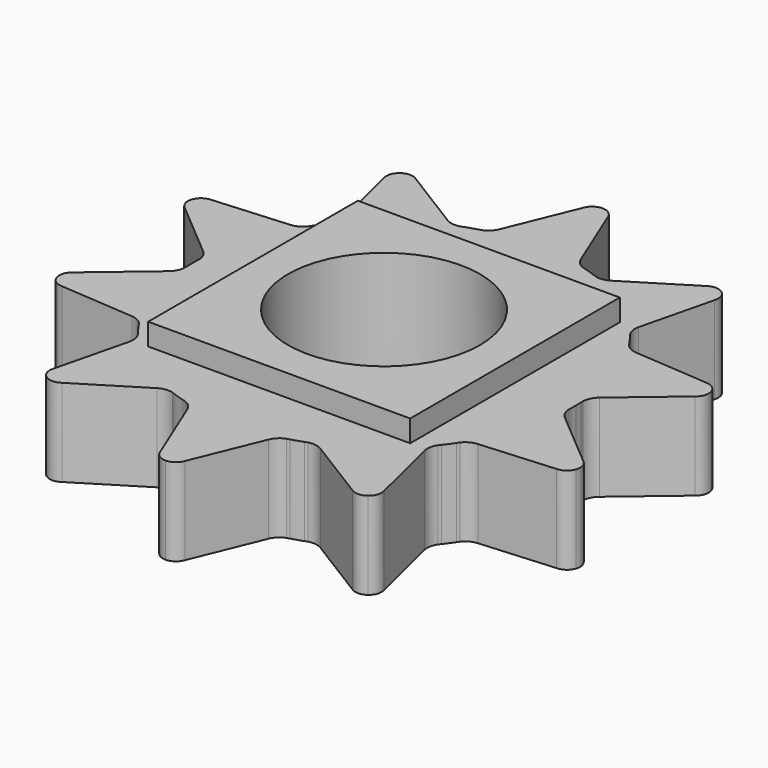
from build123d import *

# Parameters (mm, degrees)
F1_DEPTH        = 1
F1_COPIES_COUNT = 10
F3_W            = 3
F3_H            = 3
F4_DEPTH        = 0.25
F5_DEPTH        = 1
F6_DEPTH        = 0.25
F7_R            = 1.1
F8_DEPTH        = 12.5


# Not quite as in the source:
# - ends of sketch curves that miss each other by under 0.0002 mm in the source are joined
# - a feature of the source that left no trace in its solid (it failed there, or was rolled back) is left out
# - a pattern or mirror of a feature is missing from the dataset's text; its kind, count and spacing are read off the source's solid


with BuildPart() as f1:
    # F0 (on Top) → F1 (new body)
    with BuildSketch(Plane.XY):
        with BuildLine():
            ThreePointArc((0.581444512, 2.1217733808), (0.2933415776, 2.1803556405), (0, 2.2))
            ThreePointArc((0, 2.2), (-0.2933416878, 2.1803556256), (-0.5814447265, 2.121773322))
            ThreePointArc((-0.5814447265, 2.121773322), (-0.5968372157, 2.1167523736), (-0.6125853979, 2.1129929319))
            ThreePointArc((-0.6125853979, 2.1129929319), (-1.3214219849, -1.7589326132), (2.2, 0))
            ThreePointArc((2.2, 0), (1.7589325969, 1.3214220066), (0.612585346, 2.112992947))
            ThreePointArc((0.6125853416, 2.1129929319), (0.5968370782, 2.1167523965), (0.581444512, 2.1217733808))
        make_face()
        with BuildLine():
            ThreePointArc((0.6, 0.8), (0, -1), (-0.6, 0.8))
            Line((-0.6, 0.8), (0, 0.8))
            Line((0, 0.8), (0.6, 0.8))
        make_face(mode=Mode.SUBTRACT)
        with BuildLine():
            ThreePointArc((-0.5814447265, 2.121773322), (-0.2933416878, 2.1803556256), (0, 2.2))
            Line((0, 2.2), (0, 2.8273255734))
            ThreePointArc((0, 2.8273255734), (-0.1215931939, 2.889819495), (-0.1419835484, 3.0250031792))
            Line((-0.1419835484, 3.0250031792), (-0.4660251262, 2.233467269))
            ThreePointArc((-0.4660251262, 2.233467269), (-0.5120300634, 2.1655250062), (-0.5814447265, 2.121773322))
        make_face()
        with BuildLine():
            Line((0, 2.8273255734), (0, 2.2))
            ThreePointArc((0, 2.2), (0.2933415776, 2.1803556405), (0.581444512, 2.1217733808))
            ThreePointArc((0.581444512, 2.1217733808), (0.5119904355, 2.165563311), (0.4659834267, 2.2335690598))
            Line((0.4659834267, 2.2335690598), (0.1424618925, 3.0249932315))
            ThreePointArc((0.1424618925, 3.0249932315), (0.1482808399, 3.0014743175), (0.1502375048, 2.9773253853))
            ThreePointArc((0.1502375048, 2.9773253853), (0.1062195181, 2.8711754307), (0, 2.8273255734))
        make_face()
        with BuildLine():
            ThreePointArc((-0.1419835484, 3.0250031792), (-0.1215931939, 2.889819495), (0, 2.8273255734))
            Line((0, 2.8273255734), (0, 3.1273251973))
            ThreePointArc((0, 3.1273251973), (-0.0874611784, 3.0990173775), (-0.1419835484, 3.0250031792))
        make_face()
        with BuildLine():
            Line((0, 3.1273251973), (0, 2.8273255734))
            ThreePointArc((0, 2.8273255734), (0.1062195181, 2.8711754307), (0.1502375048, 2.9773253853))
            ThreePointArc((0.1502375048, 2.9773253853), (0.1482808399, 3.0014743175), (0.1424618925, 3.0249932315))
            ThreePointArc((0.1424618925, 3.0249932315), (0.0877476558, 3.0991530237), (0, 3.1273251973))
        make_face()
        with BuildLine():
            ThreePointArc((0.612585346, 2.112992947), (0.5970310708, 2.1174404125), (0.581444512, 2.1217733808))
            ThreePointArc((0.581444512, 2.1217733808), (0.5968370782, 2.1167523965), (0.6125853416, 2.1129929319))
        make_face()
        with BuildLine():
            ThreePointArc((-0.6125853979, 2.1129929319), (-0.5968372157, 2.1167523736), (-0.5814447265, 2.121773322))
            ThreePointArc((-0.5814447265, 2.121773322), (-0.5970312038, 2.117440375), (-0.6125853979, 2.1129929319))
        make_face()
    extrude(amount=F1_DEPTH)

    # F1_copies: F1 ×10 about axis
    f1_copies_axis = Axis((0, 0, 0), (0, 0, 1))


with BuildPart() as f1_1:
    add(f1.part)
    for i in range(1, F1_COPIES_COUNT):
        add(f1.part.rotate(f1_copies_axis, i * 360 / F1_COPIES_COUNT))

    # F3 (on face) → F4 (cut)
    with BuildSketch(Plane.XY.offset(1)):
        Rectangle(F3_W, F3_H)
    extrude(amount=-F4_DEPTH, mode=Mode.SUBTRACT)

    # F0 (on Top) → F5 (join)
    with BuildSketch(Plane.XY):
        with BuildLine():
            ThreePointArc((0.581444512, 2.1217733808), (0.2933415776, 2.1803556405), (0, 2.2))
            ThreePointArc((0, 2.2), (-0.2933416878, 2.1803556256), (-0.5814447265, 2.121773322))
            ThreePointArc((-0.5814447265, 2.121773322), (-0.5968372157, 2.1167523736), (-0.6125853979, 2.1129929319))
            ThreePointArc((-0.6125853979, 2.1129929319), (-1.3214219849, -1.7589326132), (2.2, 0))
            ThreePointArc((2.2, 0), (1.7589325969, 1.3214220066), (0.612585346, 2.112992947))
            ThreePointArc((0.6125853416, 2.1129929319), (0.5968370782, 2.1167523965), (0.581444512, 2.1217733808))
        make_face()
        with BuildLine():
            ThreePointArc((0.6, 0.8), (0, -1), (-0.6, 0.8))
            Line((-0.6, 0.8), (0, 0.8))
            Line((0, 0.8), (0.6, 0.8))
        make_face(mode=Mode.SUBTRACT)
        with BuildLine():
            ThreePointArc((-0.5814447265, 2.121773322), (-0.2933416878, 2.1803556256), (0, 2.2))
            Line((0, 2.2), (0, 2.8273255734))
            ThreePointArc((0, 2.8273255734), (-0.1215931939, 2.889819495), (-0.1419835484, 3.0250031792))
            Line((-0.1419835484, 3.0250031792), (-0.4660251262, 2.233467269))
            ThreePointArc((-0.4660251262, 2.233467269), (-0.5120300634, 2.1655250062), (-0.5814447265, 2.121773322))
        make_face()
        with BuildLine():
            Line((0, 2.8273255734), (0, 2.2))
            ThreePointArc((0, 2.2), (0.2933415776, 2.1803556405), (0.581444512, 2.1217733808))
            ThreePointArc((0.581444512, 2.1217733808), (0.5119904355, 2.165563311), (0.4659834267, 2.2335690598))
            Line((0.4659834267, 2.2335690598), (0.1424618925, 3.0249932315))
            ThreePointArc((0.1424618925, 3.0249932315), (0.1482808399, 3.0014743175), (0.1502375048, 2.9773253853))
            ThreePointArc((0.1502375048, 2.9773253853), (0.1062195181, 2.8711754307), (0, 2.8273255734))
        make_face()
        with BuildLine():
            ThreePointArc((-0.1419835484, 3.0250031792), (-0.1215931939, 2.889819495), (0, 2.8273255734))
            Line((0, 2.8273255734), (0, 3.1273251973))
            ThreePointArc((0, 3.1273251973), (-0.0874611784, 3.0990173775), (-0.1419835484, 3.0250031792))
        make_face()
        with BuildLine():
            Line((0, 3.1273251973), (0, 2.8273255734))
            ThreePointArc((0, 2.8273255734), (0.1062195181, 2.8711754307), (0.1502375048, 2.9773253853))
            ThreePointArc((0.1502375048, 2.9773253853), (0.1482808399, 3.0014743175), (0.1424618925, 3.0249932315))
            ThreePointArc((0.1424618925, 3.0249932315), (0.0877476558, 3.0991530237), (0, 3.1273251973))
        make_face()
        with BuildLine():
            ThreePointArc((0.612585346, 2.112992947), (0.5970310708, 2.1174404125), (0.581444512, 2.1217733808))
            ThreePointArc((0.581444512, 2.1217733808), (0.5968370782, 2.1167523965), (0.6125853416, 2.1129929319))
        make_face()
        with BuildLine():
            ThreePointArc((-0.6125853979, 2.1129929319), (-0.5968372157, 2.1167523736), (-0.5814447265, 2.121773322))
            ThreePointArc((-0.5814447265, 2.121773322), (-0.5970312038, 2.117440375), (-0.6125853979, 2.1129929319))
        make_face()
    extrude(amount=F5_DEPTH)

    # F3 (on face) → F6 (join)
    with BuildSketch(Plane.XY.offset(1)):
        Rectangle(F3_W, F3_H)
        Polygon((-0.259935757, 0.8), (0.259935757, 0.8), (0.6805206467, 0.494427191), (0.8411697794, 0), (0.6805206467, -0.494427191), (0.259935757, -0.8), (-0.259935757, -0.8), (-0.6805206467, -0.494427191), (-0.8411697794, 0), (-0.6805206467, 0.494427191), align=None, mode=Mode.SUBTRACT)
    extrude(amount=F6_DEPTH)

    # F7 (on face) → F8 (cut, symmetric)
    with BuildSketch(Plane.XY.offset(1)):
        Circle(F7_R)
    extrude(amount=F8_DEPTH, both=True, mode=Mode.SUBTRACT)


solid = f1_1.part
